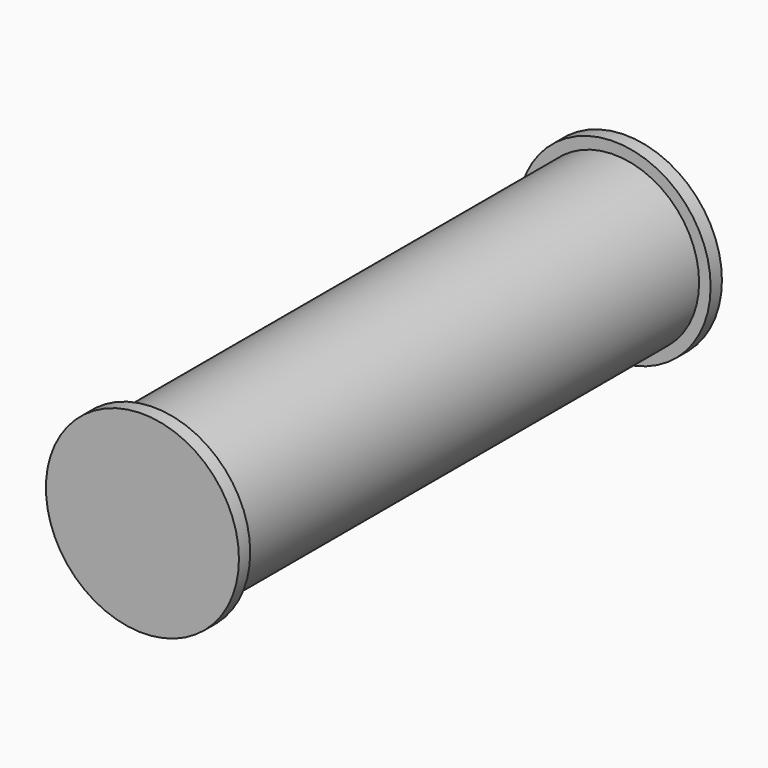
from build123d import *

# Parameters (mm, degrees)
F0_R          = 1.5303057729
F1_DEPTH      = 5.1816
F1_DEPTH_BACK = 5.1816
F2_R          = 1.7379746904
F3_DEPTH      = 0.254


# Not quite as in the source:
# - a pattern or mirror of a feature is missing from the dataset's text; its kind, count and spacing are read off the source's solid


with BuildPart() as f1:
    # F0 (on Front) → F1 (new body, two sides)
    with BuildSketch(Plane.XZ) as f1_sk:
        Circle(F0_R)
    extrude(amount=F1_DEPTH)
    extrude(f1_sk.sketch, amount=-F1_DEPTH_BACK)

    # F2 (on face) → F3 (join)
    with BuildSketch(Plane.XZ.offset(5.1816)):
        Circle(F2_R)
    f3 = extrude(amount=F3_DEPTH)

    # F3_copies: F3 across plane
    add(f3.mirror(Plane.ZX))


solid = f1.part
